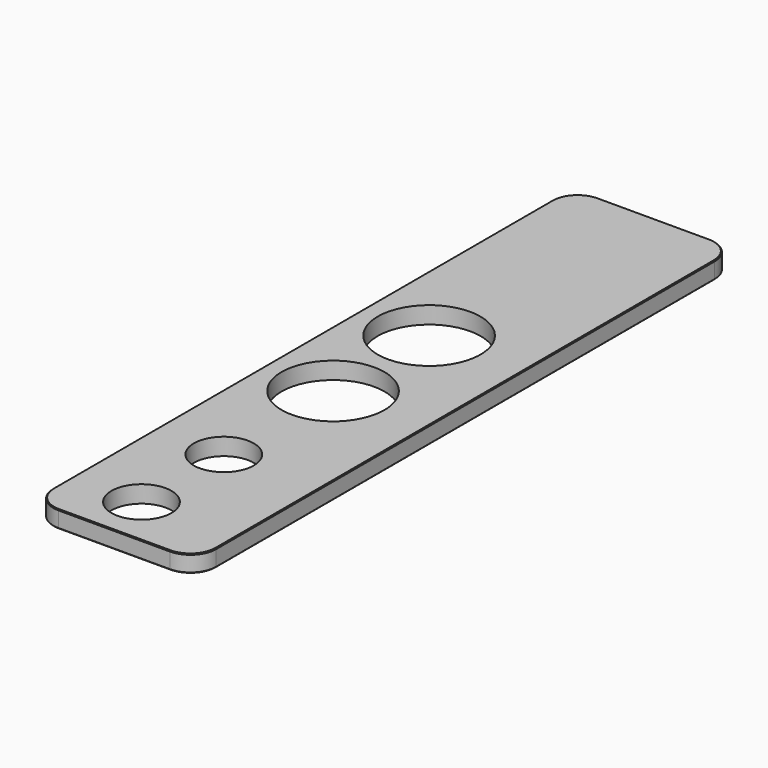
from build123d import *

# Parameters (mm, degrees)
F1_DEPTH = 1
F3_D     = 3.5
F5_D     = 6
F6_SIZE  = 0.05


with BuildPart() as f1:
    # F0 (on Top) → F1 (new body)
    with BuildSketch(Plane.XY):
        with BuildLine():
            Line((0, 37.85), (0, 1.5))
            ThreePointArc((0, 1.5), (0.4393398282, 0.4393398282), (1.5, 0))
            Line((1.5, 0), (8, 0))
            ThreePointArc((8, 0), (9.0606601718, 0.4393398282), (9.5, 1.5))
            Line((9.5, 1.5), (9.5, 37.85))
            ThreePointArc((9.5, 37.85), (9.0606601718, 38.9106601718), (8, 39.35))
            Line((8, 39.35), (1.5, 39.35))
            ThreePointArc((1.5, 39.35), (0.4393398282, 38.9106601718), (0, 37.85))
        make_face()
    extrude(amount=-F1_DEPTH)

    # F3 (through all)
    with Locations(Plane.XY):
        with Locations((3.992, 8.943), (3.992, 2.943)):
            Hole(F3_D / 2)

    # F5 (through all)
    with Locations(Plane.XY):
        with Locations((3.969, 23.94), (3.969, 16.937)):
            Hole(F5_D / 2)

    # F6
    f6_edges = [f1.edges().sort_by_distance(p)[0] for p in [
        (9.5, 19.675, 0),
        (0, 19.675, 0),
        (4.75, 0, -1),
        (4.75, 0, 0),
        (9.5, 19.675, -1),
        (4.75, 39.35, 0),
        (0, 19.675, -1),
        (4.75, 39.35, -1),
        (0.43934, 38.91066, 0),
        (0.43934, 38.91066, -1),
        (0.43934, 0.43934, 0),
        (0.43934, 0.43934, -1),
        (9.06066, 38.91066, 0),
        (9.06066, 0.43934, 0),
        (9.06066, 38.91066, -1),
        (9.06066, 0.43934, -1),
    ]]
    chamfer(f6_edges, length=F6_SIZE)


solid = f1.part
